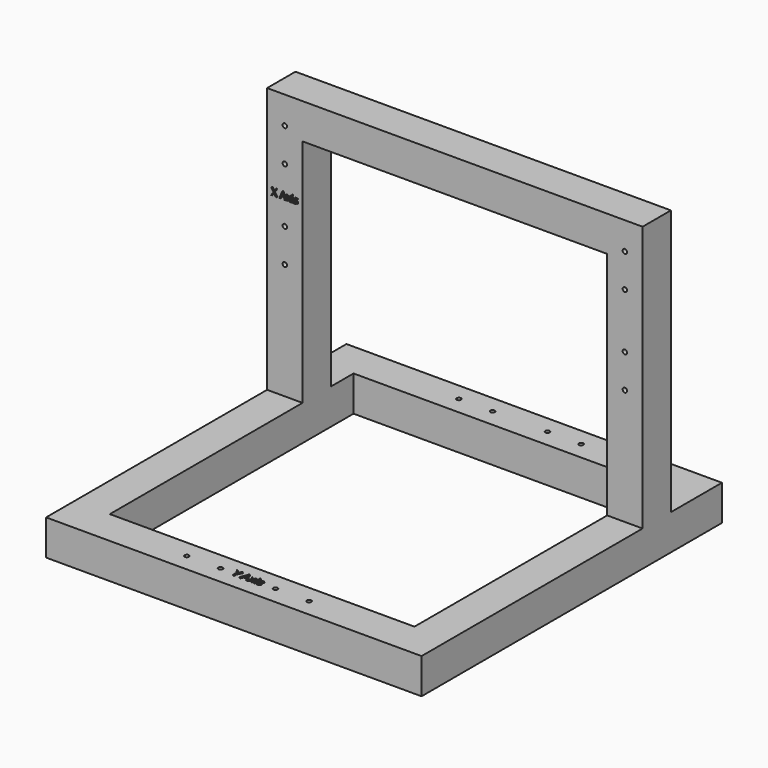
from build123d import *

# Parameters (mm, degrees)
F2_W          = 424
F2_H          = 424
F2_W_2        = 344
F2_H_2        = 344
F3_DEPTH      = 40
F4_W          = 40
F4_H          = 300
F5_DEPTH      = 40
F9_W          = 344
F9_H          = 40
F10_DEPTH     = 40
F12_D         = 5
F12_ON_F11_D  = 5
F14_TEXT_SIZE = 12.6292101211
F15_DEPTH     = 1
F13_TEXT_SIZE = 11.1697034703
F16_DEPTH     = 1


# Not quite as in the source:
# - Text() gives the source's letters only with a copy of the font that has no kerning and outlines rounded to 1/6400 em; it was checked with that copy


with BuildPart() as f3:
    # F2 (on Top) → F3 (new body)
    with BuildSketch(Plane.XY):
        Rectangle(F2_W, F2_H)
        Rectangle(F2_W_2, F2_H_2, mode=Mode.SUBTRACT)
    extrude(amount=-F3_DEPTH)

    # F7: F5 across plane


with BuildPart() as f5:
    # F4 (on Right) → F5 (new body)
    with BuildSketch(Plane.YZ):
        with Locations((120, 150)):
            Rectangle(F4_W, F4_H)
    extrude(amount=F5_DEPTH)


with BuildPart() as f5_1:
    # F6: moved
    add(f5.part.moved(Location((172, 0, 0))))


with BuildPart() as f3_1:
    add(f3.part)
    add(f5_1.part.mirror(Plane.YZ))


    add(f5_1.part)  # F10 merges F5
    # F9 (on offset) → F10 (join)
    with BuildSketch(Plane.XY.offset(300)):
        with Locations((0, 120)):
            Rectangle(F9_W, F9_H)
    extrude(amount=-F10_DEPTH)

    # F12 (through all)
    with Locations(Plane.XY):
        with Locations((-69, -192), (-31, -192), (31, -192), (69, -192), (-69, 192), (-31, 192), (31, 192), (69, 192)):
            Hole(F12_D / 2)

    # F12 on F11 (through all)
    with Locations(Plane(origin=(0, 140, 0), x_dir=(-1, 0, 0), z_dir=(0, 1, 0))):
        with Locations((-192, 269), (-192, 231), (-192, 169), (-192, 131), (192, 269), (192, 231), (192, 169), (192, 131)):
            Hole(F12_ON_F11_D / 2)

    # F14 (on face) → F15 (join)
    with BuildSketch(Plane.XY):
        with Locations((-16.7223215103, -195.8173215389)):
            Text('Y Axis', F14_TEXT_SIZE, font='Open Sans', text_align=(TextAlign.LEFT, TextAlign.BOTTOM))
    extrude(amount=F15_DEPTH)

    # F13 (on face) → F16 (join)
    with BuildSketch(Plane.XZ.offset(-100)):
        with Locations((-206.7397087812, 195.4843401909)):
            Text('X Axis', F13_TEXT_SIZE, font='Open Sans', text_align=(TextAlign.LEFT, TextAlign.BOTTOM))
    extrude(amount=F16_DEPTH)


solid = f3_1.part
